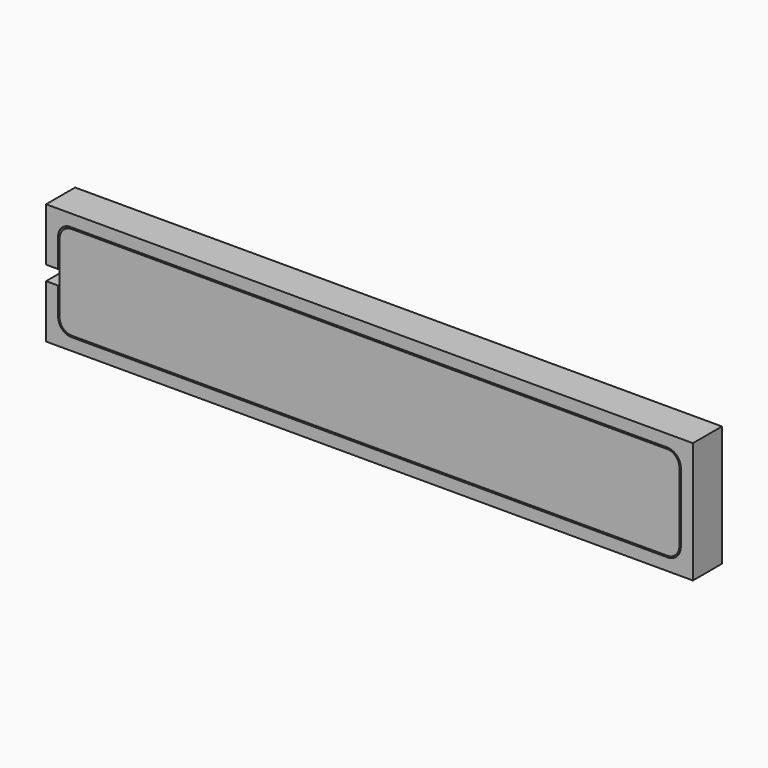
from build123d import *

# Parameters (mm, degrees)
F0_W     = 339.725
F0_H     = 63.5
F1_DEPTH = 19.05
F3_DEPTH = 12.7
F5_DEPTH = 8.89
F7_DEPTH = 7.62
F8_W     = 299.085
F8_H     = 6.604
F9_DEPTH = 25.4


with BuildPart() as f1:
    # F0 (on Front) → F1 (new body)
    with BuildSketch(Plane.XZ):
        with Locations((169.8625, 31.75)):
            Rectangle(F0_W, F0_H)
    extrude(amount=F1_DEPTH)

    # F2 (on face) → F3 (cut)
    with BuildSketch(Plane.XZ.offset(19.05)):
        with BuildLine():
            Line((313.563, 44.45), (13.462, 44.45))
            ThreePointArc((13.462, 44.45), (8.4330565722, 42.3669434278), (6.35, 37.338))
            Line((6.35, 37.338), (6.35, 35.56))
            Line((6.35, 35.56), (0, 35.56))
            Line((0, 35.56), (0, 27.94))
            Line((0, 27.94), (6.35, 27.94))
            Line((6.35, 27.94), (6.35, 26.162))
            ThreePointArc((6.35, 26.162), (8.4330565722, 21.1330565722), (13.462, 19.05))
            Line((13.462, 19.05), (313.563, 19.05))
            ThreePointArc((313.563, 19.05), (318.5919434278, 21.1330565722), (320.675, 26.162))
            Line((320.675, 26.162), (320.675, 37.338))
            ThreePointArc((320.675, 37.338), (318.5919434278, 42.3669434278), (313.563, 44.45))
        make_face()
    extrude(amount=-F3_DEPTH, mode=Mode.SUBTRACT)

    # F4 (on face) → F5 (cut)
    with BuildSketch(Plane.XZ.offset(19.05)):
        with BuildLine():
            Line((326.263, 57.15), (12.7, 57.15))
            ThreePointArc((12.7, 57.15), (8.2098719395, 55.2901280605), (6.35, 50.8))
            Line((6.35, 50.8), (6.35, 37.338))
            ThreePointArc((6.35, 37.338), (8.4330565722, 42.3669434278), (13.462, 44.45))
            Line((13.462, 44.45), (313.563, 44.45))
            ThreePointArc((313.563, 44.45), (318.5919434278, 42.3669434278), (320.675, 37.338))
            Line((320.675, 37.338), (320.675, 26.162))
            ThreePointArc((320.675, 26.162), (318.5919434278, 21.1330565722), (313.563, 19.05))
            Line((313.563, 19.05), (13.462, 19.05))
            ThreePointArc((13.462, 19.05), (8.4330565722, 21.1330565722), (6.35, 26.162))
            Line((6.35, 26.162), (6.35, 13.462))
            ThreePointArc((6.35, 13.462), (8.4330565722, 8.4330565722), (13.462, 6.35))
            Line((13.462, 6.35), (326.263, 6.35))
            ThreePointArc((326.263, 6.35), (331.2919434278, 8.4330565722), (333.375, 13.462))
            Line((333.375, 13.462), (333.375, 50.038))
            ThreePointArc((333.375, 50.038), (331.2919434278, 55.0669434278), (326.263, 57.15))
        make_face()
    extrude(amount=-F5_DEPTH, mode=Mode.SUBTRACT)

    # F8 (on face) → F9 (cut)
    with BuildSketch(Plane(origin=(0, 0, 0), x_dir=(-1, 0, 0), z_dir=(0, 1, 0))):
        with Locations((-169.8625, 31.75)):
            Rectangle(F8_W, F8_H)
    extrude(amount=-F9_DEPTH, mode=Mode.SUBTRACT)


with BuildPart() as f7:
    # F6 (on face) → F7 (new body)
    with BuildSketch(Plane.XZ.offset(19.05)):
        with BuildLine():
            Line((326.263, 56.388), (13.462, 56.388))
            ThreePointArc((13.462, 56.388), (8.9718719395, 54.5281280605), (7.112, 50.038))
            Line((7.112, 50.038), (7.112, 13.462))
            ThreePointArc((7.112, 13.462), (8.9718719395, 8.9718719395), (13.462, 7.112))
            Line((13.462, 7.112), (326.263, 7.112))
            ThreePointArc((326.263, 7.112), (330.7531280605, 8.9718719395), (332.613, 13.462))
            Line((332.613, 13.462), (332.613, 50.038))
            ThreePointArc((332.613, 50.038), (330.7531280605, 54.5281280605), (326.263, 56.388))
        make_face()
    extrude(amount=-F7_DEPTH)


solid = Compound([f1.part, f7.part])
